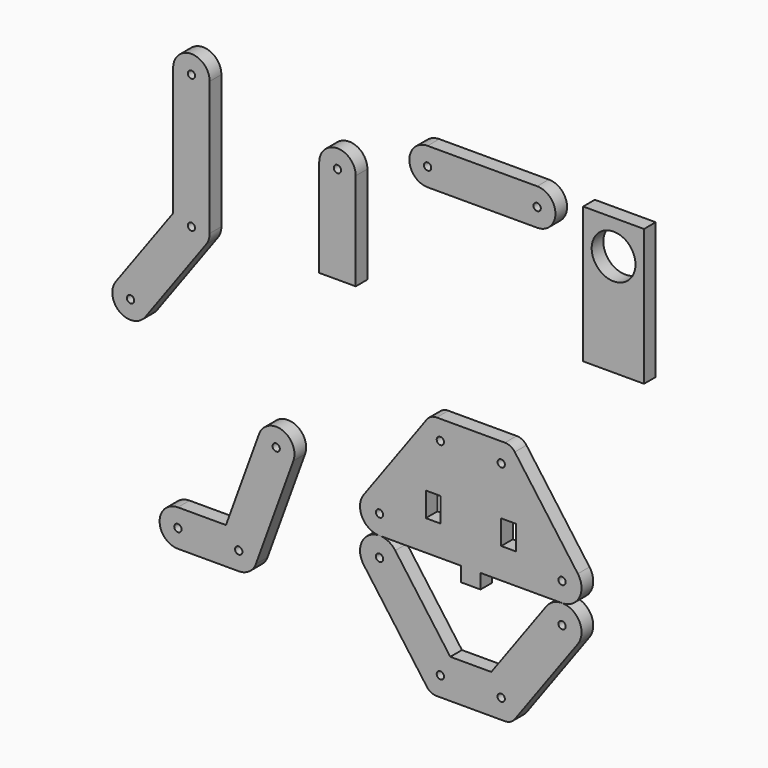
from build123d import *

# Parameters (mm, degrees)
F0_R     = 1.5
F1_DEPTH = 6
F0_W     = 25
F0_H     = 56
F0_R_2   = 9
F0_W_2   = 6
F0_H_2   = 10
F2_DEPTH = 6


with BuildPart() as f1:
    # F0 (on Front) → F1 (new body)
    with BuildSketch(Plane.XZ):
        with BuildLine():
            ThreePointArc((-105.687267783, 31.8136496476), (-104.6201626586, 33.9058026246), (-104.2524414969, 36.2254143535))
            Line((-104.2524414969, 36.2254143535), (-104.2524414969, 91.2254143535))
            ThreePointArc((-104.2524414969, 91.2254143535), (-111.7524414969, 98.7254143535), (-119.2524414969, 91.2254143535))
            Line((-119.2524414969, 91.2254143535), (-119.2524414969, 38.6646190399))
            Line((-119.2524414969, 38.6646190399), (-142.8176152108, 6.2678613472))
            ThreePointArc((-142.8176152108, 6.2678613472), (-141.1642062028, -4.2090770726), (-130.687267783, -2.5556680645))
            Line((-130.687267783, -2.5556680645), (-105.687267783, 31.8136496476))
        make_face()
        with Locations((-136.7524414969, 1.8560966413)):
            Circle(F0_R, mode=Mode.SUBTRACT)
        with Locations((-111.7524414969, 36.2254143535)):
            Circle(F0_R, mode=Mode.SUBTRACT)
        with Locations((-111.7524414969, 91.2254143535)):
            Circle(F0_R, mode=Mode.SUBTRACT)
    extrude(amount=F1_DEPTH)


with BuildPart() as f1b:
    # F0 (on Front) → F1, piece 2 (new body)
    with BuildSketch(Plane.XZ):
        with BuildLine():
            ThreePointArc((-44.2505994937, 76.5896396789), (-51.7505994937, 84.0896396789), (-59.2505994937, 76.5896396789))
            Line((-59.2505994937, 76.5896396789), (-59.2505994937, 36.5896396789))
            Line((-59.2505994937, 36.5896396789), (-44.2505994937, 36.5896396789))
            Line((-44.2505994937, 36.5896396789), (-44.2505994937, 76.5896396789))
        make_face()
        with Locations((-51.7505994937, 76.5896396789)):
            Circle(F0_R, mode=Mode.SUBTRACT)
    extrude(amount=F1_DEPTH)


with BuildPart() as f1c:
    # F0 (on Front) → F1, piece 3 (new body)
    with BuildSketch(Plane.XZ):
        with BuildLine():
            ThreePointArc((-14.7224422544, 97.0328903141), (-22.2224422544, 89.5328903141), (-14.7224422544, 82.0328903141))
            Line((-14.7224422544, 82.0328903141), (30.2775577456, 82.0328903141))
            ThreePointArc((30.2775577456, 82.0328903141), (37.7775577456, 89.5328903141), (30.2775577456, 97.0328903141))
            Line((30.2775577456, 97.0328903141), (-14.7224422544, 97.0328903141))
        make_face()
        with Locations((-14.7224422544, 89.5328903141)):
            Circle(F0_R, mode=Mode.SUBTRACT)
        with Locations((30.2775577456, 89.5328903141)):
            Circle(F0_R, mode=Mode.SUBTRACT)
    extrude(amount=F1_DEPTH)


with BuildPart() as f1d:
    # F0 (on Front) → F1, piece 4 (new body)
    with BuildSketch(Plane.XZ):
        with BuildLine():
            ThreePointArc((-69.8688708126, -34.8479340648), (-74.3514143936, -25.2350883339), (-83.9642601244, -29.7176319149))
            Line((-83.9642601244, -29.7176319149), (-97.5590284548, -67.0689509252))
            Line((-97.5590284548, -67.0689509252), (-117.3074719182, -67.0689509252))
            ThreePointArc((-117.3074719182, -67.0689509252), (-124.8074719182, -74.5689509252), (-117.3074719182, -82.0689509252))
            Line((-117.3074719182, -82.0689509252), (-92.3074719182, -82.0689509252))
            ThreePointArc((-92.3074719182, -82.0689509252), (-88.0056486456, -80.7125912574), (-85.2597772623, -77.1341020002))
            Line((-85.2597772623, -77.1341020002), (-69.8688708126, -34.8479340648))
        make_face()
        with Locations((-117.3074719182, -74.5689509252)):
            Circle(F0_R, mode=Mode.SUBTRACT)
        with Locations((-92.3074719182, -74.5689509252)):
            Circle(F0_R, mode=Mode.SUBTRACT)
        with Locations((-76.9165654685, -32.2827829898)):
            Circle(F0_R, mode=Mode.SUBTRACT)
    extrude(amount=F1_DEPTH)


with BuildPart() as f1e:
    # F0 (on Front) → F1, piece 5 (new body)
    with BuildSketch(Plane.XZ):
        with Locations((61.6822957993, 67.8637354374)):
            Rectangle(F0_W, F0_H)
        with Locations((61.6822957993, 81.8637354374)):
            Circle(F0_R_2, mode=Mode.SUBTRACT)
    extrude(amount=F1_DEPTH)


with BuildPart() as f1f:
    # F0 (on Front) → F1, piece 6 (new body)
    with BuildSketch(Plane.XZ):
        with BuildLine():
            ThreePointArc((-28.0125484861, -53.6634353592), (-30.8521262624, -51.2402554027), (-34.4820671142, -50.3693177122))
            ThreePointArc((-34.4820671142, -50.3693177122), (-41.6111294237, -54.7393768603), (-40.9515857424, -63.0752000651))
            Line((-40.9515857424, -63.0752000651), (-15.0530414885, -98.6798118949))
            ThreePointArc((-15.0530414885, -98.6798118949), (-13.2783053783, -100.1942993677), (-11.0095923459, -100.7386354243))
            Line((-11.0095923459, -100.7386354243), (3.0179328858, -100.7386354243))
            Line((3.0179328858, -100.7386354243), (17.0454581174, -100.7386354243))
            ThreePointArc((17.0454581174, -100.7386354243), (19.3141711498, -100.1942993677), (21.08890726, -98.6798118949))
            Line((21.08890726, -98.6798118949), (46.9874515139, -63.0752000651))
            ThreePointArc((46.9874515139, -63.0752000651), (47.6469951952, -54.7393768603), (40.5179328858, -50.3693177122))
            ThreePointArc((40.5179328858, -50.3693177122), (36.8879920339, -51.2402554027), (34.0484142576, -53.6634353592))
            Line((34.0484142576, -53.6634353592), (11.444532268, -84.7386354243))
            Line((11.444532268, -84.7386354243), (3.0179328858, -84.7386354243))
            Line((3.0179328858, -84.7386354243), (-5.4086664965, -84.7386354243))
            Line((-5.4086664965, -84.7386354243), (-28.0125484861, -53.6634353592))
        make_face()
        with Locations((-9.4820671142, -92.7386354243)):
            Circle(F0_R, mode=Mode.SUBTRACT)
        with Locations((-34.4820671142, -58.3693177122)):
            Circle(F0_R, mode=Mode.SUBTRACT)
        with Locations((15.5179328858, -92.7386354243)):
            Circle(F0_R, mode=Mode.SUBTRACT)
        with Locations((40.5179328858, -58.3693177122)):
            Circle(F0_R, mode=Mode.SUBTRACT)
    extrude(amount=F1_DEPTH)


with BuildPart() as f2:
    # F0 (on Front) → F2 (new body)
    with BuildSketch(Plane.XZ):
        with BuildLine():
            Line((17.0454581174, 0), (3.0179328858, 0))
            Line((3.0179328858, 0), (-11.0095923459, 0))
            ThreePointArc((-11.0095923459, 0), (-13.2783053783, -0.5443360566), (-15.0530414885, -2.0588235294))
            Line((-15.0530414885, -2.0588235294), (-40.9515857424, -37.6634353592))
            ThreePointArc((-40.9515857424, -37.6634353592), (-41.6111294237, -45.9992585641), (-34.4820671142, -50.3693177122))
            Line((-34.4820671142, -50.3693177122), (-0.9820671142, -50.3693177122))
            Line((-0.9820671142, -50.3693177122), (-0.9820671142, -56.3693177122))
            Line((-0.9820671142, -56.3693177122), (7.0179328858, -56.3693177122))
            Line((7.0179328858, -56.3693177122), (7.0179328858, -50.3693177122))
            Line((7.0179328858, -50.3693177122), (40.5179328858, -50.3693177122))
            ThreePointArc((40.5179328858, -50.3693177122), (47.6469951952, -45.9992585641), (46.9874515139, -37.6634353592))
            Line((46.9874515139, -37.6634353592), (21.08890726, -2.0588235294))
            ThreePointArc((21.08890726, -2.0588235294), (19.3141711498, -0.5443360566), (17.0454581174, 0))
        make_face()
        with Locations((-34.4820671142, -42.3693177122)):
            Circle(F0_R, mode=Mode.SUBTRACT)
        with Locations((-12.4820671142, -32.8693177122)):
            Rectangle(F0_W_2, F0_H_2, mode=Mode.SUBTRACT)
        with Locations((-9.4820671142, -8)):
            Circle(F0_R, mode=Mode.SUBTRACT)
        with Locations((18.5179328858, -32.8693177122)):
            Rectangle(F0_W_2, F0_H_2, mode=Mode.SUBTRACT)
        with Locations((40.5179328858, -42.3693177122)):
            Circle(F0_R, mode=Mode.SUBTRACT)
        with Locations((15.5179328858, -8)):
            Circle(F0_R, mode=Mode.SUBTRACT)
    extrude(amount=F2_DEPTH)


solid = Compound([f1.part, f1b.part, f1c.part, f1d.part, f1e.part, f1f.part, f2.part])
